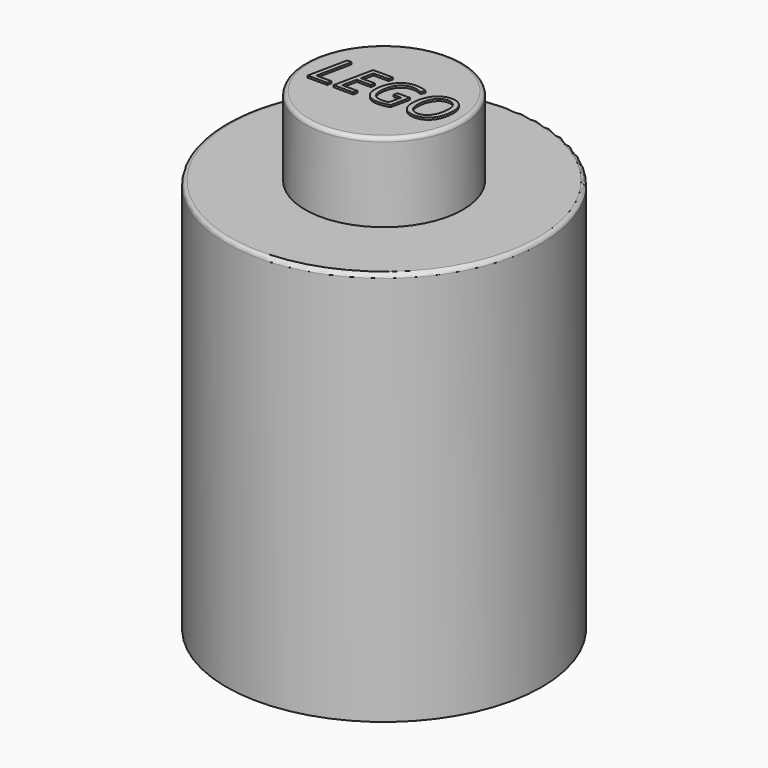
from build123d import *

# Parameters (mm, degrees)
F0_R         = 8
F1_DEPTH     = 20
F2_R         = 4
F3_DEPTH     = 4
F4_T         = -2
F5_R         = 0.2
F6_TEXT_SIZE = 2.7777777778
F7_DEPTH     = 0.1


# Not quite as in the source:
# - Text() gives the source's letters only with a copy of the font that has no kerning and outlines rounded to 1/6400 em; it was checked with that copy


with BuildPart() as f1:
    # F0 (on Top) → F1 (new body)
    with BuildSketch(Plane.XY):
        with Locations((-8, 0)):
            Circle(F0_R)
    extrude(amount=F1_DEPTH)

    # F2 (on face) → F3 (join)
    with BuildSketch(Plane.XY.offset(20)):
        with Locations((-8, 0)):
            Circle(F2_R)
    extrude(amount=F3_DEPTH)

    # F4
    f4_openings = [f1.faces().sort_by_distance(p)[0] for p in [
        (-8, 0, 0),
    ]]
    offset(amount=F4_T, openings=f4_openings, kind=Kind.INTERSECTION)

    # F5
    f5_edges = [f1.edges().sort_by_distance(p)[0] for p in [
        (-16, 0, 20),
        (-12, 0, 24),
    ]]
    fillet(f5_edges, radius=F5_R)

    # F6 (on face) → F7 (join)
    with BuildSketch(Plane.XY.offset(24)):
        with Locations((-11.1898348859, -1.0042044511)):
            Text('LEGO', F6_TEXT_SIZE, font='Open Sans', font_style=FontStyle.ITALIC, text_align=(TextAlign.LEFT, TextAlign.BOTTOM))
    extrude(amount=F7_DEPTH)


solid = f1.part
